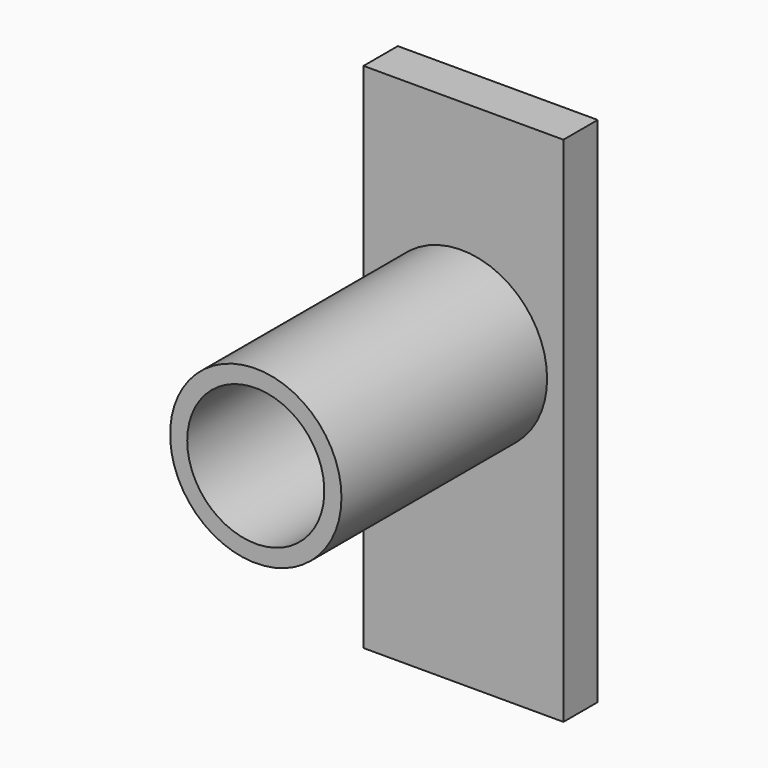
from build123d import *

# Parameters (mm, degrees)
F0_R      = 7.62
F1_DEPTH  = 22.86
F2_R      = 5.3975
F3_DEPTH  = 25.4
F4_W      = 17.78
F4_H      = 45.5848994723
F5_DEPTH  = 3.81
F6_DEPTH  = 25.4
F7_R      = 6.0983154317
F8_DEPTH  = 25.4
F9_R      = 3.7193661061
F10_DEPTH = 17.78
F11_DEPTH = 25.4


with BuildPart() as f1:
    # F0 (on Front) → F1 (new body)
    with BuildSketch(Plane.XZ):
        with Locations((-16.9606450945, 18.8963711262)):
            Circle(F0_R)
    extrude(amount=F1_DEPTH)

    # F2 (on face) → F3 (cut)
    with BuildSketch(Plane.XZ.offset(22.86)):
        with Locations((-16.9606450945, 18.8963711262)):
            Circle(F2_R)
    extrude(amount=-F3_DEPTH, mode=Mode.SUBTRACT)

    # F4 (on Front) → F5 (join)
    with BuildSketch(Plane.XZ):
        with Locations((-16.7762902565, 15.3014517855)):
            Rectangle(F4_W, F4_H)
    extrude(amount=-F5_DEPTH)

    # F6 (cut): a face of the model
    f6_faces = [f1.faces().sort_by_distance(p)[0] for p in [
        (-16.9606450945, 0, 18.8963711262),
    ]]
    extrude(f6_faces, amount=-F6_DEPTH, mode=Mode.SUBTRACT)

    # F7 (on face) → F8 (cut)
    with BuildSketch(Plane(origin=(0, 3.81, 0), x_dir=(-1, 0, 0), z_dir=(0, 1, 0))):
        with Locations((16.9606450945, 18.8963711262)):
            Circle(F7_R)
    extrude(amount=-F8_DEPTH, mode=Mode.SUBTRACT)

    # F9 (on Top) → F10 (cut)
    with BuildSketch(Plane.XY):
        with Locations((-17.3269938678, -7.0897382684)):
            Circle(F9_R)
    extrude(amount=F10_DEPTH, mode=Mode.SUBTRACT)

    # F11 (cut): a face of the model
    f11_faces = [f1.faces().sort_by_distance(p)[0] for p in [
        (-11.0348160706, -21.59, 18.8963711262),
    ]]
    extrude(f11_faces, amount=-F11_DEPTH, mode=Mode.SUBTRACT)


solid = f1.part
